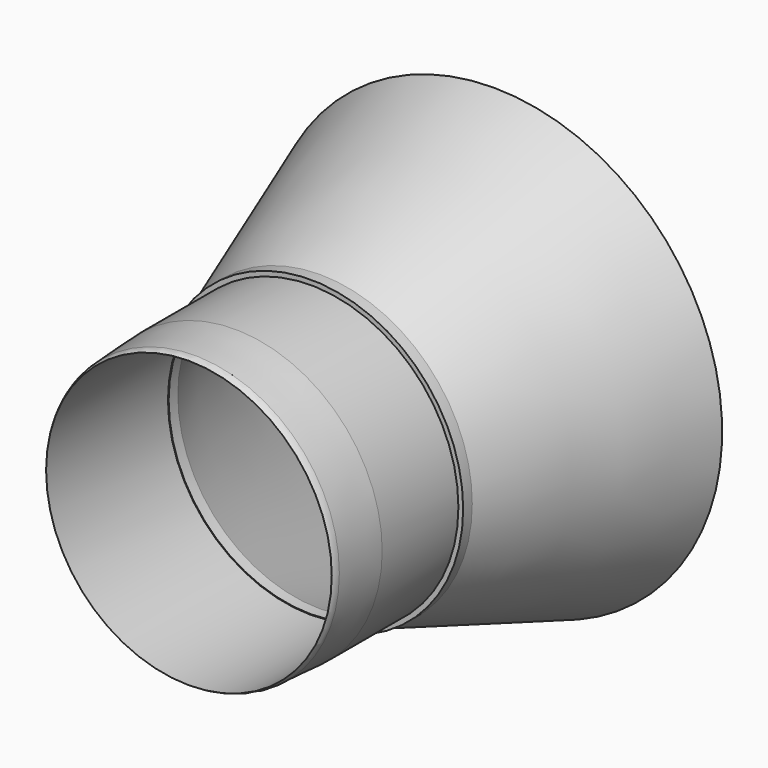
from build123d import *

# Parameters (mm, degrees)
F0_R          = 50.8
F0_R_2        = 47.625
F1_DEPTH      = 3.81
F1_DEPTH_BACK = 50.8
F2_R          = 50.8
F2_R_2        = 49.2125
F3_DEPTH      = 50.801
F4_SIZE2      = 1.016
F4_SIZE       = 19.05


# Not quite as in the source:
# - a fillet or chamfer that OpenCascade refuses, or shapes differently, is made with other operations: its cross-section is extruded or revolved along the edge and cut away or added


with BuildPart() as f1:
    # F0 (on Front) → F1 (new body, two sides)
    with BuildSketch(Plane.XZ) as f1_sk:
        Circle(F0_R)
        Circle(F0_R_2, mode=Mode.SUBTRACT)
    extrude(amount=-F1_DEPTH)
    extrude(f1_sk.sketch, amount=F1_DEPTH_BACK)

    # F2 (on Front) → F3 (cut, through all)
    with BuildSketch(Plane.XZ):
        Circle(F2_R)
        Circle(F2_R_2, mode=Mode.SUBTRACT)
    extrude(amount=F3_DEPTH, mode=Mode.SUBTRACT)

    # F4
    f4_edges = [f1.edges().sort_by_distance(p)[0] for p in [
        (-49.2125, -50.8, 0),
    ]]
    chamfer(f4_edges, length=F4_SIZE, length2=F4_SIZE2)

    # F5: fillet of radius 5.08 on 1 edges, made by hand

    # F5_s1 → F5_t2 (revolve, cut)
    with BuildSketch(Plane.XY):
        with BuildLine():
            ThreePointArc((48.3194667684, -48.4943730928), (48.1108173968, -49.6889287689), (47.625, -50.8))
            Line((47.625, -50.8), (48.1965, -50.8))
            Line((48.1965, -50.8), (48.3194667684, -48.4943730928))
        make_face()
    revolve(axis=Axis((0, -50.8, 0), (0, 1, 0)), mode=Mode.SUBTRACT)

    # F6 (on Right) → F7 (revolve)
    with BuildSketch(Plane.YZ):
        Polygon((76.2, 76.2), (3.81, 50.8), (0, 50.8), (0, 47.407604754), (3.81, 47.407604754), (60.2590404451, 67.3254877329), align=None)
    revolve(axis=Axis((0, 38.1, 0), (0, -1, 0)))


solid = f1.part
